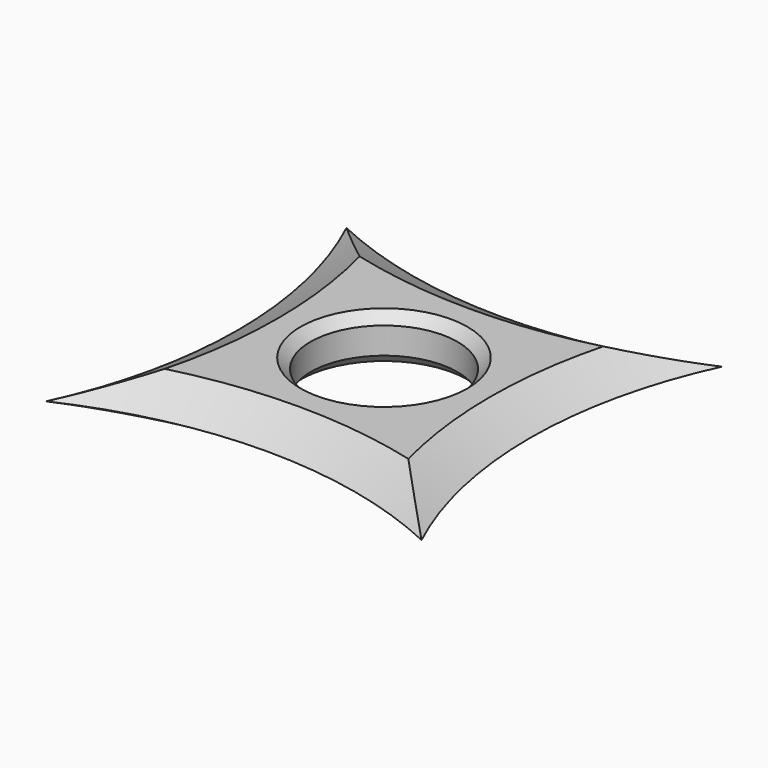
from build123d import *

# Parameters (mm, degrees)
F0_R     = 11.075
F1_DEPTH = 7
F2_SIZE2 = 6
F2_SIZE  = 3.5
F3_SIZE2 = 3.49999
F3_SIZE  = 5.99999
F4_SIZE  = 1.5


# Not quite as in the source:
# - a fillet or chamfer is up to 0.001 mm smaller than in the source, because OpenCascade refuses the exact size


with BuildPart() as f1:
    # F0 (on Top) → F1 (new body)
    with BuildSketch(Plane.XY):
        with BuildLine():
            ThreePointArc((28.2842712475, -28.2842712475), (21.9994915516, 0), (28.2842712475, 28.2842712475))
            ThreePointArc((28.2842712475, 28.2842712475), (0, 21.9994915516), (-28.2842712475, 28.2842712475))
            ThreePointArc((-28.2842712475, 28.2842712475), (-21.9994915516, 0), (-28.2842712475, -28.2842712475))
            ThreePointArc((-28.2842712475, -28.2842712475), (0, -21.9994915516), (28.2842712475, -28.2842712475))
        make_face()
        Circle(F0_R, mode=Mode.SUBTRACT)
    extrude(amount=F1_DEPTH)

    # F2
    f2_edges = [f1.edges().sort_by_distance(p)[0] for p in [
        (0, -21.999492, 7),
        (-21.999492, 0, 7),
        (0, 21.999492, 7),
        (21.999492, 0, 7),
    ]]
    chamfer(f2_edges, length=F2_SIZE, length2=F2_SIZE2)

    # F3 (size 6 and 3.5 in the source; OpenCascade refuses exactly that, so slightly less here)
    f3_edges = [f1.edges().sort_by_distance(p)[0] for p in [
        (-21.999492, 0, 0),
        (0, -21.999492, 0),
        (21.999492, 0, 0),
        (0, 21.999492, 0),
    ]]
    f3_side = f1.faces().sort_by_distance((0, -21.199492, 0))[0]
    chamfer(f3_edges, length=F3_SIZE, length2=F3_SIZE2, reference=f3_side)

    # F4
    f4_edges = [f1.edges().sort_by_distance(p)[0] for p in [
        (-11.075, 0, 0),
        (-11.075, 0, 7),
    ]]
    chamfer(f4_edges, length=F4_SIZE)


solid = f1.part
